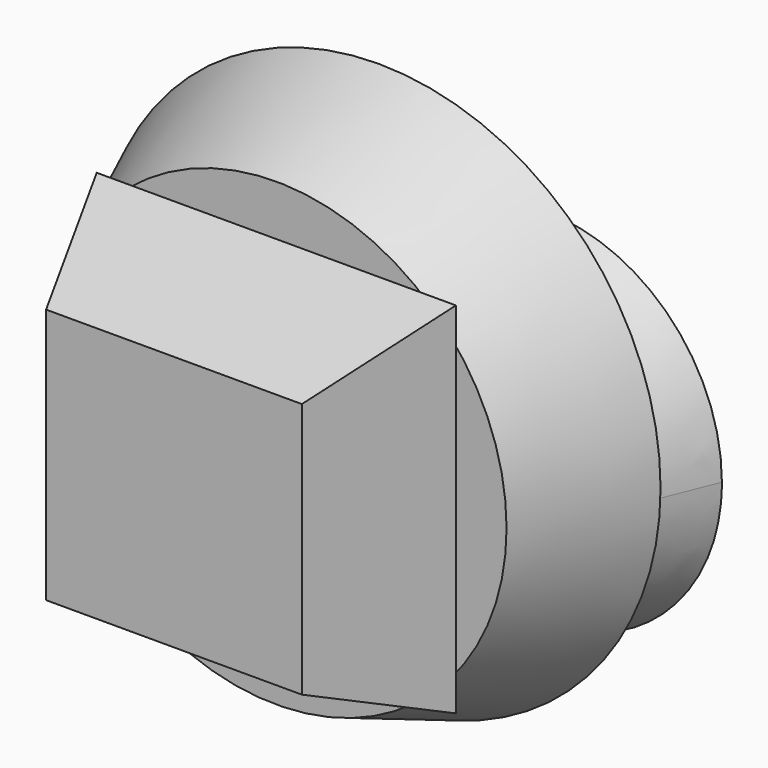
from build123d import *

# Parameters (mm, degrees)
F2_W     = 150
F2_H     = 150
F5_DEPTH = 75
F5_TAPER = -22
F3_R     = 135.0187980494


with BuildPart() as f5:
    # F2 (on offset) → F5 (new body)
    with BuildSketch(Plane.XZ.offset(75)):
        Rectangle(F2_W, F2_H)
    extrude(amount=-F5_DEPTH, taper=F5_TAPER)


with BuildPart() as f5b:
    # F3 (on Front) → F5, piece 2 (new body)
    with BuildSketch(Plane.XZ):
        Circle(F3_R)
    extrude(amount=-F5_DEPTH, taper=F5_TAPER)


with BuildPart() as f5c:
    # F4 (on offset) → F5, piece 3 (new body)
    with BuildSketch(Plane.XZ.offset(-75)):
        with BuildLine():
            add(Edge.make_bspline(
                [(-35.3803634644, -35.2156162262), (-35.3803634644, -166.5215816961), (74.4028091431, -100.8685989611), (184.1859817505, -35.2156162262), (74.4028091431, 30.4373665087), (-35.3803634644, 96.0903492437), (-35.3803634644, -35.2156162262)],
                knots=[4.7123889804, 4.7123889804, 4.7123889804, 6.8067840828, 6.8067840828, 8.9011791852, 8.9011791852, 10.9955742876, 10.9955742876, 10.9955742876], degree=2, weights=[1, 0.5, 1, 0.5, 1, 0.5, 1]))
        make_face()
    extrude(amount=-F5_DEPTH, taper=F5_TAPER)


solid = Compound([f5.part, f5b.part, f5c.part])
